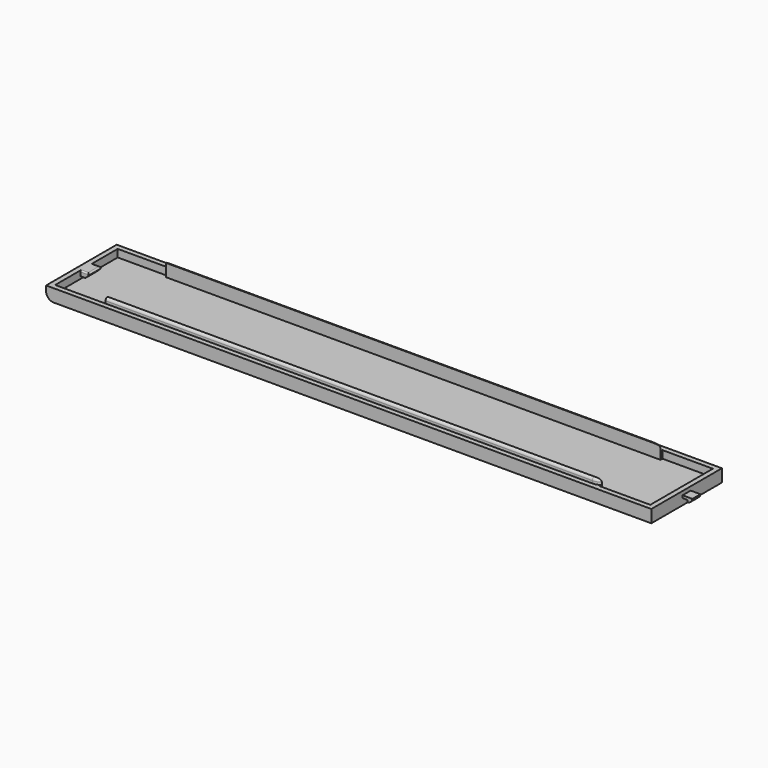
from build123d import *

# Parameters (mm, degrees)
F0_W         = 35
F0_H         = 5
F1_DEPTH     = 120
F2_T         = -2
F4_DEPTH     = 3
F6_DEPTH     = 2
F7_T1_DEPTH  = 10.0971618345
F8_W         = 196
F8_H         = 5
F9_DEPTH     = 1
F10_W        = 196
F10_H        = 2
F10_H_2      = 3
F11_DEPTH    = 1
F12_T1_DEPTH = 9.5
F13_R        = 0.99999
F14_R        = 0.5
F15_R        = 4
F16_DEPTH    = 1
F17_W        = 2
F17_H        = 10
F18_DEPTH    = 1
F19_R        = 0.99999
F20_R        = 3


# Not quite as in the source:
# - a fillet or chamfer that OpenCascade refuses, or shapes differently, is made with other operations: its cross-section is extruded or revolved along the edge and cut away or added
# - a fillet or chamfer is up to 0.001 mm smaller than in the source, because OpenCascade refuses the exact size


with BuildPart() as f1:
    # F0 (on Right) → F1 (new body, symmetric)
    with BuildSketch(Plane.YZ):
        Rectangle(F0_W, F0_H)
    extrude(amount=F1_DEPTH, both=True)

    # F2
    f2_openings = [f1.faces().sort_by_distance(p)[0] for p in [
        (0, 0, 2.5),
    ]]
    offset(amount=F2_T, openings=f2_openings)

    # F3 (on Front) → F4 (join, symmetric)
    with BuildSketch(Plane.XZ):
        Polygon((-114, 2.5), (-118, 2.5), (-118, 0.5), (-116, 0.5), align=None)
    extrude(amount=F4_DEPTH, both=True)

    # F5 (on Front) → F6 (join, symmetric)
    with BuildSketch(Plane.XZ):
        Polygon((123.9, 1), (120, 1), (120, 0), (121.9, 0), (123.9, 0), align=None)
        Polygon((121.9, -1), (123.9, 0), (121.9, 0), align=None)
    extrude(amount=F6_DEPTH, both=True)

    # F7: fillet of radius 2 on 1 edges, made by hand

    # F7_s2 → F7_t1 (cut)
    with BuildSketch(Plane.XZ.offset(-5.0485809173)):
        with BuildLine():
            ThreePointArc((123.9, 1), (123.5488845703, 0.09023972), (122.8093065335, -0.5453467333))
            Line((122.8093065335, -0.5453467333), (123.9, 0))
            Line((123.9, 0), (123.9, 1))
        make_face()
    extrude(amount=F7_T1_DEPTH, mode=Mode.SUBTRACT)

    # F8 (on face) → F9 (join)
    with BuildSketch(Plane(origin=(0, -15.5, 0), x_dir=(-1, 0, 0), z_dir=(0, 1, 0))):
        with Locations((0, 2)):
            Rectangle(F8_W, F8_H)
    extrude(amount=F9_DEPTH)

    # F10 (on face) → F11 (join)
    with BuildSketch(Plane.XZ.offset(-15.5)):
        with Locations((0, 3.5)):
            Rectangle(F10_W, F10_H)
        with Locations((0, 1)):
            Rectangle(F10_W, F10_H_2)
    extrude(amount=F11_DEPTH)

    # F12: fillet of radius 5 on 2 edges, made by hand

    # F12_s2 → F12_t1 (cut)
    with BuildSketch(Plane.XY.offset(2.5)):
        with BuildLine():
            ThreePointArc((95, 15.5), (96.5811388301, 15.2434164903), (98, 14.5))
            Line((98, 14.5), (98, 15.5))
            Line((98, 15.5), (95, 15.5))
        make_face()
        with BuildLine():
            ThreePointArc((95, -15.5), (96.5811388301, -15.2434164903), (98, -14.5))
            Line((98, -14.5), (98, -15.5))
            Line((98, -15.5), (95, -15.5))
        make_face()
    extrude(amount=F12_T1_DEPTH, mode=Mode.SUBTRACT)

    # F13 (radius 1 in the source; OpenCascade refuses exactly that, so slightly less here)
    f13_edges = [f1.edges().sort_by_distance(p)[0] for p in [
        (-1.5, -15.5, 4.5),
        (-1.5, 15.5, 4.5),
    ]]
    fillet(f13_edges, radius=F13_R)

    # F14
    f14_edges = [f1.edges().sort_by_distance(p)[0] for p in [
        (-114, 0, 2.5),
        (-116, -3, 2.5),
        (-116, 3, 2.5),
    ]]
    fillet(f14_edges, radius=F14_R)

    # F15 (on face) → F16 (cut)
    with BuildSketch(Plane(origin=(0, 0, -2.5), x_dir=(1, 0, 0), z_dir=(0, 0, -1))):
        with Locations((-107, 11.5)):
            Circle(F15_R)
        with Locations((-107, -11.5)):
            Circle(F15_R)
        with Locations((112, -11.5)):
            Circle(F15_R)
        with Locations((112, 11.5)):
            Circle(F15_R)
    extrude(amount=-F16_DEPTH, mode=Mode.SUBTRACT)

    # F17 (on face) → F18 (join)
    with BuildSketch(Plane(origin=(0, 0, -2.5), x_dir=(1, 0, 0), z_dir=(0, 0, -1))):
        with Locations((114, 0)):
            Rectangle(F17_W, F17_H)
    extrude(amount=F18_DEPTH)

    # F19 (radius 1 in the source; OpenCascade refuses exactly that, so slightly less here)
    f19_edges = [f1.edges().sort_by_distance(p)[0] for p in [
        (114, -5, -3.5),
        (115, 0, -3.5),
        (114, 5, -3.5),
        (113, 0, -3.5),
    ]]
    fillet(f19_edges, radius=F19_R)

    # F20
    f20_edges = [f1.edges().sort_by_distance(p)[0] for p in [
        (-120, 0, -2.5),
    ]]
    fillet(f20_edges, radius=F20_R)


solid = f1.part
